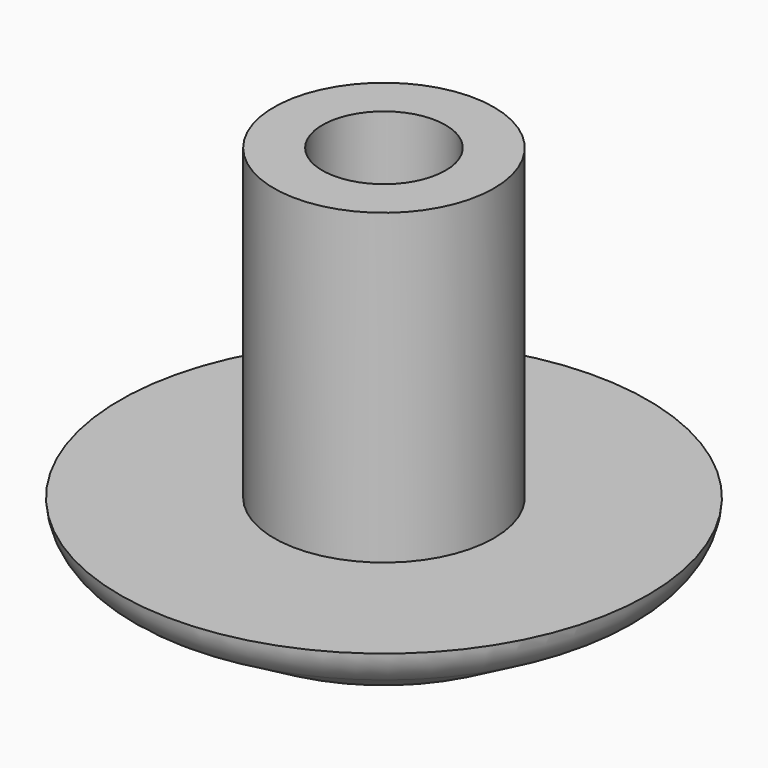
from build123d import *

# Parameters (mm, degrees)
F0_R     = 6
F1_DEPTH = 2
F2_SIZE2 = 2.5980762114
F2_SIZE  = 1.5
F4_R     = 2.5
F4_R_2   = 1.4
F5_DEPTH = 7
F6_R     = 1.2


# Not quite as in the source:
# - a fillet or chamfer that OpenCascade refuses, or shapes differently, is made with other operations: its cross-section is extruded or revolved along the edge and cut away or added


with BuildPart() as f1:
    # F0 (on Top) → F1 (new body)
    with BuildSketch(Plane.XY):
        Circle(F0_R)
    extrude(amount=F1_DEPTH)

    # F2
    f2_edges = [f1.edges().sort_by_distance(p)[0] for p in [
        (-6, 0, 0),
    ]]
    f2_side = f1.faces().sort_by_distance((-6, 0, 1))[0]
    chamfer(f2_edges, length=F2_SIZE, length2=F2_SIZE2, reference=f2_side)

    # F3: fillet of radius 1 on 2 edges, made by hand

    # F3_s1 → F3_t2 (revolve, cut)
    with BuildSketch(Plane.XZ):
        with BuildLine():
            ThreePointArc((3.6339745962, 0.1339745962), (3.3927936413, 0.0340741737), (3.1339745962, 0))
            Line((3.1339745962, 0), (3.4019237886, 0))
            Line((3.4019237886, 0), (3.6339745962, 0.1339745962))
        make_face()
    revolve(axis=Axis((0, 0, 0), (0, 0, 1)), mode=Mode.SUBTRACT)

    # F3_s3 → F3_t4 (revolve, cut)
    with BuildSketch(Plane.XZ):
        with BuildLine():
            ThreePointArc((6, 2), (5.8486778537, 1.5452494356), (5.5031382462, 1.2131367327))
            Line((5.5031382462, 1.2131367327), (6, 1.5))
            Line((6, 1.5), (6, 2))
        make_face()
    revolve(axis=Axis((0, 0, 1.5), (0, 0, 1)), mode=Mode.SUBTRACT)

    # F4 (on face) → F5 (join)
    with BuildSketch(Plane.XY.offset(2)):
        Circle(F4_R)
        Circle(F4_R_2, mode=Mode.SUBTRACT)
    extrude(amount=F5_DEPTH)

    # F6
    f6_edges = [f1.edges().sort_by_distance(p)[0] for p in [
        (-1.4, 0, 2),
    ]]
    fillet(f6_edges, radius=F6_R)


solid = f1.part
